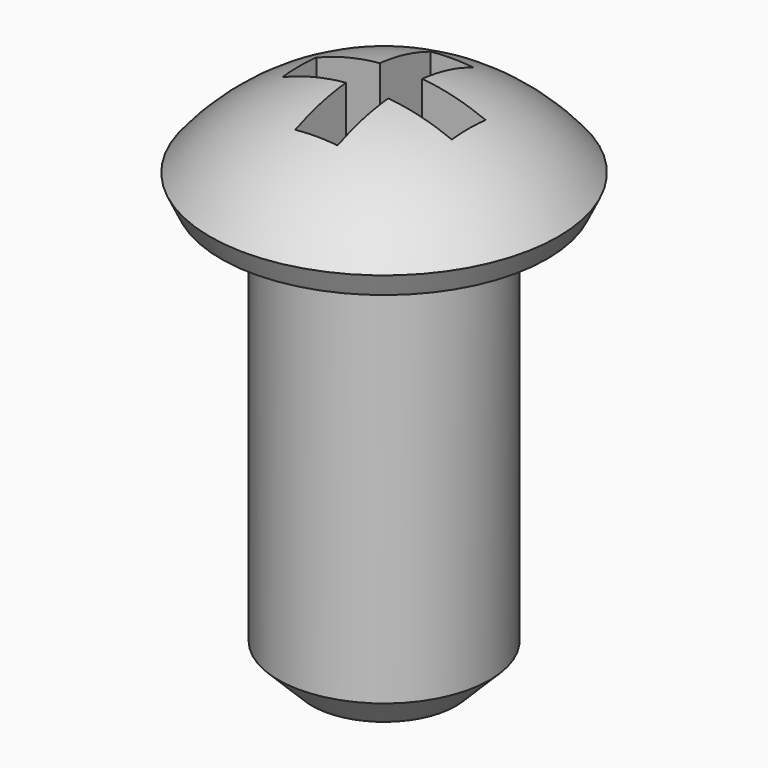
from build123d import *

# Parameters (mm, degrees)
F4_DEPTH = 3.176
F5_SIZE  = 1.016


# Not quite as in the source:
# - a fillet or chamfer that OpenCascade refuses, or shapes differently, is made with other operations: its cross-section is extruded or revolved along the edge and cut away or added


with BuildPart() as f1:
    # F0 (on Front) → F1 (revolve)
    with BuildSketch(Plane.XZ):
        with BuildLine():
            Line((3.175, 0), (5.715, 0))
            ThreePointArc((5.715, 0), (3.2688625698, 2.3279526256), (0, 3.175))
            Line((0, 3.175), (0, -12.7))
            Line((0, -12.7), (3.175, -12.7))
            Line((3.175, -12.7), (3.175, 0))
        make_face()
    revolve(axis=Axis((0, 0, -4.7625), (0, 0, 1)))

    # F2: chamfer of 0.762 on 1 edges, made by hand

    # F2_s1 → F2_t2 (revolve, cut)
    with BuildSketch(Plane.XZ):
        with BuildLine():
            Line((4.8809391349, -0.0275238998), (5.2355867217, 0.7179265843))
            Line((5.2355867217, 0.7179265843), (5.2474112325, 0.727541081))
            ThreePointArc((5.2474112325, 0.727541081), (5.4877257432, 0.3678527374), (5.7279396226, 0.0080513208))
            Line((5.7279396226, 0.0080513208), (5.715, -0.01524))
            ThreePointArc((5.715, -0.01524), (5.2979695675, -0.01524), (4.8809391349, -0.0427638998))
            Line((4.8809391349, -0.0427638998), (4.8809391349, -0.0275238998))
        make_face()
    revolve(axis=Axis((0, 0, 0), (0, 0, 1)), mode=Mode.SUBTRACT)

    # F3 (on Top) → F4 (cut, through all)
    with BuildSketch(Plane.XY):
        Polygon((0.635, 2.54), (-0.635, 2.54), (-0.635, 0.635), (-2.54, 0.635), (-2.54, -0.635), (-0.635, -0.635), (-0.635, -2.54), (0.635, -2.54), (0.635, -0.635), (2.54, -0.635), (2.54, 0.635), (0.635, 0.635), align=None)
    extrude(amount=F4_DEPTH, mode=Mode.SUBTRACT)

    # F5
    f5_edges = [f1.edges().sort_by_distance(p)[0] for p in [
        (-3.175, 0, -12.7),
    ]]
    chamfer(f5_edges, length=F5_SIZE)


solid = f1.part
